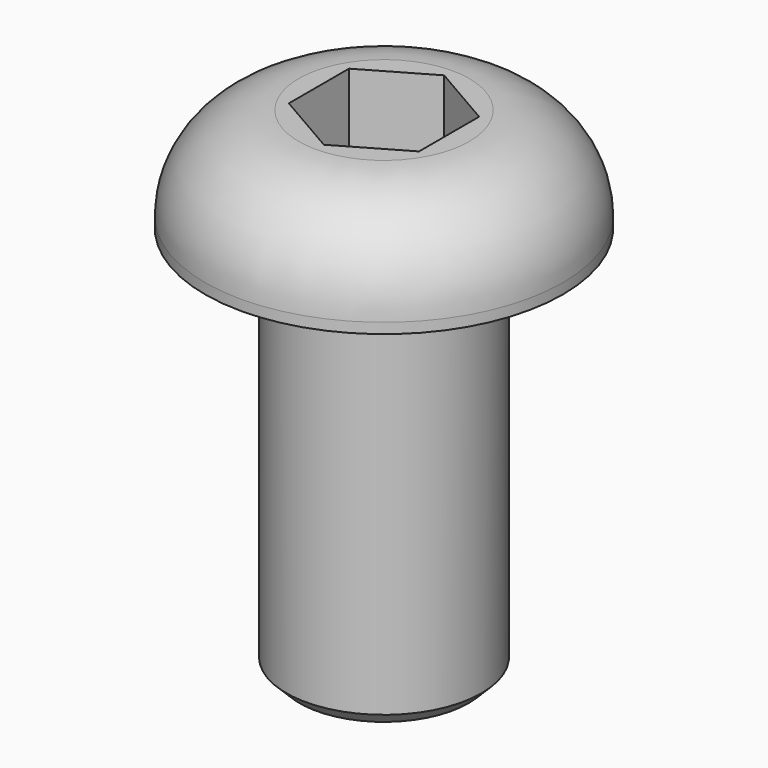
from build123d import *

# Parameters (mm, degrees)
F3_DEPTH = 1.6
F6_SIZE  = 0.2


# Not quite as in the source:
# - an extrude whose draft closes it to a point is written as a loft to that point


with BuildPart() as f1:
    # F0 (on Front) → F1 (revolve)
    with BuildSketch(Plane.XZ):
        with BuildLine():
            Line((0, 1.6), (0, -6))
            Line((0, -6), (1.5, -6))
            Line((1.5, -6), (1.5, 0))
            Line((1.5, 0), (2.75, 0))
            Line((2.75, 0), (2.75, 0.16))
            ThreePointArc((2.75, 0.16), (2.3282337649, 1.1782337649), (1.31, 1.6))
            Line((1.31, 1.6), (0, 1.6))
        make_face()
    revolve(axis=Axis((0, 0, 3.7619129732), (0, 0, 1)))

    # F2 (on face) → F3 (cut)
    with BuildSketch(Plane.XY.offset(1.6)):
        Polygon((-1, 0.5773502692), (-1, -0.5773502692), (0, -1.1547005384), (1, -0.5773502692), (1, 0.5773502692), (0, 1.1547005384), align=None)
    extrude(amount=-F3_DEPTH, mode=Mode.SUBTRACT)

    # F4 (on face) → F5 section 0
    with BuildSketch(Plane.XY, mode=Mode.PRIVATE) as f5_s0:
        Polygon((-1, 0.5773502692), (-1, -0.5773502692), (0, -1.1547005384), (1, -0.5773502692), (1, 0.5773502692), (0, 1.1547005384), align=None)
    loft([f5_s0.sketch, Vertex(0, 0, -0.3639702343)], ruled=True, mode=Mode.SUBTRACT)

    # F6
    f6_edges = [f1.edges().sort_by_distance(p)[0] for p in [
        (-1.5, 0, -6),
    ]]
    chamfer(f6_edges, length=F6_SIZE)


solid = f1.part
